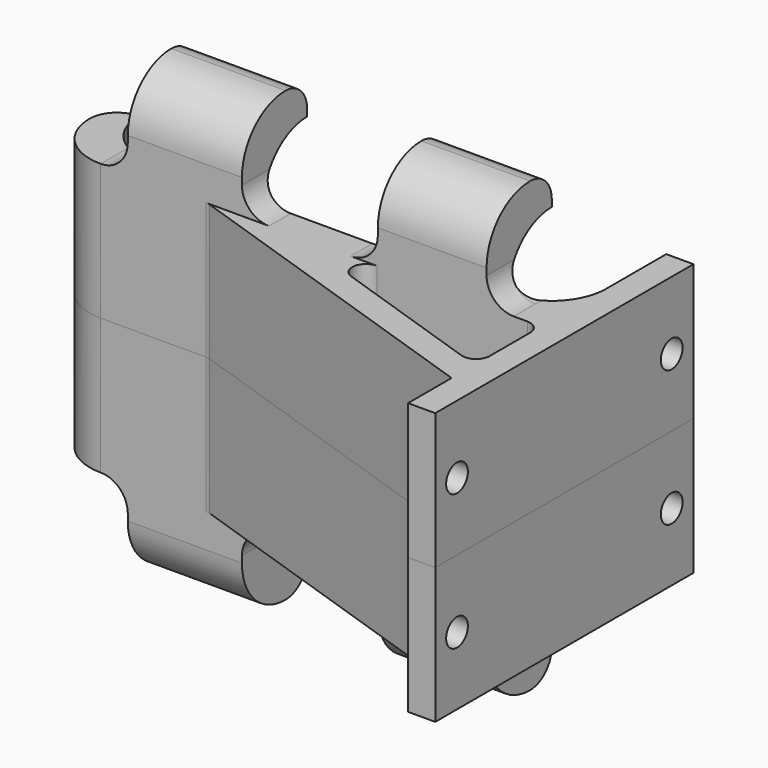
from build123d import *

# Parameters (mm, degrees)
F1_DEPTH      = 25
F2_R          = 2.5
F3_DEPTH      = 25
F4_R          = 4.99999
F5_R          = 2.5
F7_START      = -15
F7_DEPTH      = 20
F8_START      = -60
F8_DEPTH      = 21
F9_R          = 4.99999
F10_T4_DEPTH  = 17.5
F10_S5_R      = 10
F10_T6_DEPTH  = 11
F10_T10_DEPTH = 17.5
F10_S11_R     = 10
F10_T12_DEPTH = 11
F10_T16_DEPTH = 17.5
F10_S17_R     = 10
F10_T18_DEPTH = 11
F10_T22_DEPTH = 30
F10_S23_R     = 10
F10_T24_DEPTH = 17
F10_T29_DEPTH = 17.5
F10_S30_R     = 10
F10_T31_DEPTH = 11
F10_T35_DEPTH = 17.5
F10_S36_R     = 10
F10_T37_DEPTH = 11
F10_T38_DEPTH = 45


# Not quite as in the source:
# - a fillet or chamfer that OpenCascade refuses, or shapes differently, is made with other operations: its cross-section is extruded or revolved along the edge and cut away or added
# - a fillet or chamfer is up to 0.001 mm smaller than in the source, because OpenCascade refuses the exact size


with BuildPart() as f1:
    # F0 (on Top) → F1 (new body)
    with BuildSketch(Plane.XY):
        with BuildLine():
            ThreePointArc((11.9032669473, 15), (8.9743347592, 7.9289321881), (1.9032669473, 5))
            Line((1.9032669473, 5), (-64.0967330527, 5))
            ThreePointArc((-64.0967330527, 5), (-71.1678008646, 7.9289321881), (-74.0967330527, 15))
            Line((-74.0967330527, 15), (-79.0967330527, 15))
            Line((-79.0967330527, 15), (-79.0967330527, 10))
            ThreePointArc((-79.0967330527, 10), (-76.1678008646, 2.9289321881), (-69.0967330527, 0))
            Line((-69.0967330527, 0), (-49.3079621117, 0))
            Line((-49.3079621117, 0), (11.9032669473, -20.5484238273))
            Line((11.9032669473, -20.5484238273), (11.9032669473, -30.5484238273))
            Line((11.9032669473, -30.5484238273), (16.9032669473, -30.5484238273))
            Line((16.9032669473, -30.5484238273), (16.9032669473, 15))
            Line((16.9032669473, 15), (16.9032669473, 28.8165863603))
            Line((16.9032669473, 28.8165863603), (11.9032669473, 28.8165863603))
            Line((11.9032669473, 28.8165863603), (11.9032669473, 15))
        make_face()
        Polygon((-33.5967330527, 0), (11.9032669473, 0), (11.9032669473, -15.2742119136), align=None, mode=Mode.SUBTRACT)
    extrude(amount=F1_DEPTH)

    # F2 (on face) → F3 (cut)
    with BuildSketch(Plane.YZ.offset(16.9032669473)):
        with Locations((-25.5484238273, 12.5)):
            Circle(F2_R)
        with Locations((23.8165863603, 12.5)):
            Circle(F2_R)
    extrude(amount=-F3_DEPTH, mode=Mode.SUBTRACT)

    # F4 (radius 5 in the source; OpenCascade refuses exactly that, so slightly less here)
    f4_edges = [f1.edges().sort_by_distance(p)[0] for p in [
        (-79.096733, 15, 12.5),
    ]]
    fillet(f4_edges, radius=F4_R)

    # F5
    f5_edges = [f1.edges().sort_by_distance(p)[0] for p in [
        (-33.596733, 0, 12.5),
        (11.903267, 0, 12.5),
        (11.903267, -15.274212, 12.5),
        (-49.307962, 0, 12.5),
    ]]
    fillet(f5_edges, radius=F5_R)

    # F6 (on face) → F7 (join)
    with BuildSketch(Plane.YZ.offset(16.9032669473).offset(F7_START)):
        with BuildLine():
            Line((0, 31.2271468341), (0, 25))
            Line((0, 25), (5, 25))
            ThreePointArc((5, 25), (7.9289321881, 32.0710678119), (15, 35))
            Line((15, 35), (15, 41.2271468341))
            Line((15, 41.2271468341), (10, 41.2271468341))
            ThreePointArc((10, 41.2271468341), (2.9289321881, 38.298214646), (0, 31.2271468341))
        make_face()
    extrude(amount=-F7_DEPTH)

    # F6 (on face) → F8 (join)
    with BuildSketch(Plane.YZ.offset(16.9032669473).offset(F8_START)):
        with BuildLine():
            Line((0, 31.2271468341), (0, 25))
            Line((0, 25), (5, 25))
            ThreePointArc((5, 25), (7.9289321881, 32.0710678119), (15, 35))
            Line((15, 35), (15, 41.2271468341))
            Line((15, 41.2271468341), (10, 41.2271468341))
            ThreePointArc((10, 41.2271468341), (2.9289321881, 38.298214646), (0, 31.2271468341))
        make_face()
    extrude(amount=-F8_DEPTH)

    # F9 (radius 5 in the source; OpenCascade refuses exactly that, so slightly less here)
    f9_edges = [f1.edges().sort_by_distance(p)[0] for p in [
        (-53.596733, 15, 41.227147),
    ]]
    fillet(f9_edges, radius=F9_R)

    # F10: fillet of radius 5 on 5 edges, made by hand


with BuildPart() as f10_tool2:
    # F10_s3 → F10_t4 (new body)
    with BuildSketch(Plane.XZ):
        with BuildLine():
            ThreePointArc((6.9032669473, 25), (3.3677330414, 26.4644660941), (1.9032669473, 30))
            Line((1.9032669473, 30), (1.9032669473, 25))
            Line((1.9032669473, 25), (6.9032669473, 25))
        make_face()
    extrude(amount=-F10_T4_DEPTH)

    # F10_s5 → F10_t6 (cut, symmetric)
    with BuildSketch(Plane.YZ.offset(4.4)):
        with Locations((15, 25)):
            Circle(F10_S5_R)
    extrude(amount=F10_T6_DEPTH, both=True, mode=Mode.SUBTRACT)


with BuildPart() as f1_1:
    add(f1.part)

    # F10_t1: union F10_tool2
    add(f10_tool2.part)


with BuildPart() as f10_tool8:
    # F10_s9 → F10_t10 (new body)
    with BuildSketch(Plane.XZ):
        with BuildLine():
            ThreePointArc((6.9032669473, 25), (3.3677330414, 26.4644660941), (1.9032669473, 30))
            Line((1.9032669473, 30), (1.9032669473, 25))
            Line((1.9032669473, 25), (6.9032669473, 25))
        make_face()
    extrude(amount=-F10_T10_DEPTH)

    # F10_s11 → F10_t12 (cut, symmetric)
    with BuildSketch(Plane.XY.offset(27.5)):
        with Locations((1.9032669473, 15)):
            Circle(F10_S11_R)
    extrude(amount=F10_T12_DEPTH, both=True, mode=Mode.SUBTRACT)


with BuildPart() as f1_2:
    add(f1_1.part)

    # F10_t7: union F10_tool8
    add(f10_tool8.part)


with BuildPart() as f10_tool14:
    # F10_s15 → F10_t16 (new body)
    with BuildSketch(Plane.XZ):
        with BuildLine():
            ThreePointArc((-64.0967330527, 30), (-65.5611991468, 26.4644660941), (-69.0967330527, 25))
            Line((-69.0967330527, 25), (-64.0967330527, 25))
            Line((-64.0967330527, 25), (-64.0967330527, 30))
        make_face()
    extrude(amount=-F10_T16_DEPTH)

    # F10_s17 → F10_t18 (cut, symmetric)
    with BuildSketch(Plane.XY.offset(27.5)):
        with Locations((-64.0967330527, 15)):
            Circle(F10_S17_R)
    extrude(amount=F10_T18_DEPTH, both=True, mode=Mode.SUBTRACT)


with BuildPart() as f1_3:
    add(f1_2.part)

    # F10_t13: union F10_tool14
    add(f10_tool14.part)


with BuildPart() as f10_tool20:
    # F10_s21 → F10_t22 (new body)
    with BuildSketch(Plane.XZ.offset(12.5)):
        with BuildLine():
            ThreePointArc((-64.0967330527, 30), (-65.5611991468, 26.4644660941), (-69.0967330527, 25))
            Line((-69.0967330527, 25), (-64.0967330527, 25))
            Line((-64.0967330527, 25), (-64.0967330527, 30))
        make_face()
    extrude(amount=-F10_T22_DEPTH)

    # F10_s23 → F10_t24 (cut, symmetric)
    with BuildSketch(Plane.YZ.offset(-66.6)):
        with Locations((15, 25)):
            Circle(F10_S23_R)
    extrude(amount=F10_T24_DEPTH, both=True, mode=Mode.SUBTRACT)

    split(bisect_by=Plane.XZ.offset(-5), keep=Keep.BOTTOM)


with BuildPart() as f1_4:
    add(f1_3.part)

    # F10_t19: union F10_tool20
    add(f10_tool20.part)


with BuildPart() as f10_tool27:
    # F10_s28 → F10_t29 (new body)
    with BuildSketch(Plane.XZ):
        with BuildLine():
            ThreePointArc((-43.0967330527, 30), (-41.6322669586, 26.4644660941), (-38.0967330527, 25))
            Line((-38.0967330527, 25), (-43.0967330527, 25))
            Line((-43.0967330527, 25), (-43.0967330527, 30))
        make_face()
    extrude(amount=-F10_T29_DEPTH)

    # F10_s30 → F10_t31 (cut, symmetric)
    with BuildSketch(Plane.YZ.offset(-40.6)):
        with Locations((15, 25)):
            Circle(F10_S30_R)
    extrude(amount=F10_T31_DEPTH, both=True, mode=Mode.SUBTRACT)


with BuildPart() as f1_5:
    add(f1_4.part)

    # F10_t26: union F10_tool27
    add(f10_tool27.part)


with BuildPart() as f10_tool33:
    # F10_s34 → F10_t35 (new body)
    with BuildSketch(Plane.XZ):
        with BuildLine():
            ThreePointArc((-23.0967330527, 25), (-19.5611991468, 26.4644660941), (-18.0967330527, 30))
            Line((-18.0967330527, 30), (-18.0967330527, 25))
            Line((-18.0967330527, 25), (-23.0967330527, 25))
        make_face()
    extrude(amount=-F10_T35_DEPTH)

    # F10_s36 → F10_t37 (cut, symmetric)
    with BuildSketch(Plane.YZ.offset(-20.6)):
        with Locations((15, 25)):
            Circle(F10_S36_R)
    extrude(amount=F10_T37_DEPTH, both=True, mode=Mode.SUBTRACT)


with BuildPart() as f1_6:
    add(f1_5.part)

    # F10_t32: union F10_tool33
    add(f10_tool33.part)

    # F10_s39 → F10_t38 (cut)
    with BuildSketch(Plane.YZ.offset(-30.5967330527)):
        with BuildLine():
            ThreePointArc((10, 41.2271468341), (13.5355339059, 39.7626807401), (15, 36.2271468341))
            Line((15, 36.2271468341), (15, 41.2271468341))
            Line((15, 41.2271468341), (10, 41.2271468341))
        make_face()
    extrude(amount=F10_T38_DEPTH, mode=Mode.SUBTRACT)


with BuildPart() as f11_1:
    # F11: instance of F1
    add(f1_6.part.mirror(Plane.XY))


solid = Compound([f1_6.part, f11_1.part])
